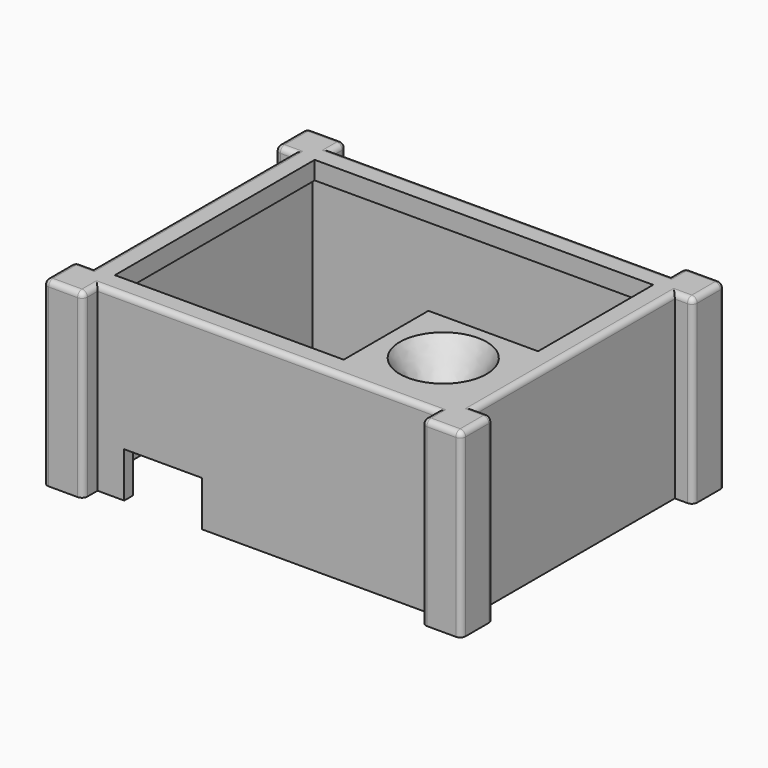
from build123d import *

# Parameters (mm, degrees)
F0_W          = 60.594435811
F0_H          = 58.5138263702
F0_R          = 27.5
F3_DEPTH      = 10
F4_R          = 5
F6_R          = 24
F7_R          = 3
F9_DEPTH      = 10
F10_DEPTH     = 100
F0_W_2        = 42.894218117
F0_H_2        = 6
F11_DEPTH     = 75
F12_R         = 3
F13_T1_DEPTH  = 104.5
F13_S5_W      = 3
F13_S5_H      = 3
F13_T6_DEPTH  = 3
F13_S11_W     = 3
F13_S11_H     = 3
F13_T12_DEPTH = 3
F13_S17_W     = 3
F13_S17_H     = 3
F13_T18_DEPTH = 3
F13_S23_W     = 3
F13_S23_H     = 3
F13_T24_DEPTH = 3
F13_S29_W     = 3
F13_S29_H     = 3
F13_T30_DEPTH = 3
F13_S35_W     = 3
F13_S35_H     = 3
F13_T36_DEPTH = 3
F13_S41_W     = 3
F13_S41_H     = 3
F13_T42_DEPTH = 3
F13_S47_W     = 3
F13_S47_H     = 3
F13_T48_DEPTH = 3
F13_S53_W     = 3
F13_S53_H     = 3
F13_T54_DEPTH = 3
F13_S59_W     = 3
F13_S59_H     = 3
F13_T60_DEPTH = 3
F13_S65_W     = 3
F13_S65_H     = 3
F13_T66_DEPTH = 3
F13_S71_W     = 3
F13_S71_H     = 3
F13_T72_DEPTH = 3
F14_SCALE     = 0.5
F15_ANGLE     = 180


# Not quite as in the source:
# - a fillet or chamfer that OpenCascade refuses, or shapes differently, is made with other operations: its cross-section is extruded or revolved along the edge and cut away or added


with BuildPart() as f3:
    # F0 (on Top) → F3 (new body)
    with BuildSketch(Plane.XY):
        with Locations((162.7266414762, 114.7430868149)):
            Rectangle(F0_W, F0_H)
        with Locations((165, 116)):
            Circle(F0_R, mode=Mode.SUBTRACT)
        with Locations((165, 116)):
            Circle(F0_R)
    extrude(amount=F3_DEPTH)

    # F4 (on offset) → F5 section 0
    with BuildSketch(Plane.XY.offset(36)):
        with Locations((165.0143116713, 116.0647049546)):
            Circle(F4_R)
    # F0 (on Top) → F5 section 1
    with BuildSketch(Plane.XY):
        with Locations((165, 116)):
            Circle(F0_R)
    loft()

    # F6 (on Top) → F8 section 0
    with BuildSketch(Plane.XY):
        with Locations((164.9883985519, 115.9429103136)):
            Circle(F6_R)
    # F7 (on offset) → F8 section 1
    with BuildSketch(Plane.XY.offset(36)):
        with Locations((164.916202426, 116.0804182291)):
            Circle(F7_R)
    loft(mode=Mode.SUBTRACT)

    # F0 (on Top) → F9 (join)
    with BuildSketch(Plane.XY):
        Polygon((0, 150), (0, 0), (199, 0), (199, 150), (63.6303052306, 150), (20.7360871136, 150), align=None)
        Polygon((193.0238593817, 6), (6, 6), (6, 144), (132.4294235706, 144), (193.0238593817, 144), (193.0238593817, 85.4861736298), align=None, mode=Mode.SUBTRACT)
    extrude(amount=F9_DEPTH)

    # F0 (on Top) → F10 (join)
    with BuildSketch(Plane.XY):
        Polygon((199, 0), (0, 0), (0, 150), (20.7360871136, 150), (20.7360871136, 156), (6, 156), (6, 166), (-16, 166), (-16, 144), (-6, 144), (-6, 6), (-16, 6), (-16, -16), (6, -16), (6, -6), (193.0238593817, -6), (193.0238593817, -16), (215, -16), (215, 6), (205, 6), (205, 144), (215, 144), (215, 166), (193.0238593817, 166), (193.0238593817, 156), (63.6303052306, 156), (63.6303052306, 150), (199, 150), align=None)
    extrude(amount=F10_DEPTH)

    # F0 (on Top) → F11 (join)
    with BuildSketch(Plane.XY):
        with Locations((42.1831961721, 153)):
            Rectangle(F0_W_2, F0_H_2)
    extrude(amount=F11_DEPTH)

    # F12
    f12_edges = [f3.edges().sort_by_distance(p)[0] for p in [
        (204.01193, -16, 0),
        (215, -5, 0),
        (205, 75, 0),
        (210, 6, 0),
        (210, 144, 0),
        (215, 155, 0),
        (204.01193, 166, 0),
        (193.023859, 161, 0),
        (99.51193, 156, 0),
        (-5, 166, 0),
        (6, 161, 0),
        (-16, 155, 0),
        (-11, 144, 0),
        (-6, 75, 0),
        (-11, 6, 0),
        (-5, -16, 0),
        (-16, -5, 0),
        (6, -11, 0),
        (99.51193, -6, 0),
        (193.023859, -11, 0),
    ]]
    fillet(f12_edges, radius=F12_R)

    # F13: fillet of radius 3 on 12 edges, made by hand

    # F13_s2 → F13_t1 (cut)
    with BuildSketch(Plane.XY.offset(3)):
        with BuildLine():
            ThreePointArc((212, -16), (214.1213203436, -15.1213203436), (215, -13))
            Line((215, -13), (215, -16))
            Line((215, -16), (212, -16))
        make_face()
        with BuildLine():
            ThreePointArc((193.0238593817, -13), (193.9025390381, -15.1213203436), (196.0238593817, -16))
            Line((196.0238593817, -16), (193.0238593817, -16))
            Line((193.0238593817, -16), (193.0238593817, -13))
        make_face()
        with BuildLine():
            ThreePointArc((215, 3), (214.1213203436, 5.1213203436), (212, 6))
            Line((212, 6), (215, 6))
            Line((215, 6), (215, 3))
        make_face()
        with BuildLine():
            ThreePointArc((212, 144), (214.1213203436, 144.8786796564), (215, 147))
            Line((215, 147), (215, 144))
            Line((215, 144), (212, 144))
        make_face()
        with BuildLine():
            ThreePointArc((215, 163), (214.1213203436, 165.1213203436), (212, 166))
            Line((212, 166), (215, 166))
            Line((215, 166), (215, 163))
        make_face()
        with BuildLine():
            ThreePointArc((193.0238593817, 163), (193.9025390381, 165.1213203436), (196.0238593817, 166))
            Line((196.0238593817, 166), (193.0238593817, 166))
            Line((193.0238593817, 166), (193.0238593817, 163))
        make_face()
        with BuildLine():
            ThreePointArc((3, -16), (5.1213203436, -15.1213203436), (6, -13))
            Line((6, -13), (6, -16))
            Line((6, -16), (3, -16))
        make_face()
        with BuildLine():
            ThreePointArc((-16, -13), (-15.1213203436, -15.1213203436), (-13, -16))
            Line((-13, -16), (-16, -16))
            Line((-16, -16), (-16, -13))
        make_face()
        with BuildLine():
            ThreePointArc((-13, 6), (-15.1213203436, 5.1213203436), (-16, 3))
            Line((-16, 3), (-16, 6))
            Line((-16, 6), (-13, 6))
        make_face()
        with BuildLine():
            ThreePointArc((-16, 147), (-15.1213203436, 144.8786796564), (-13, 144))
            Line((-13, 144), (-16, 144))
            Line((-16, 144), (-16, 147))
        make_face()
        with BuildLine():
            ThreePointArc((-13, 166), (-15.1213203436, 165.1213203436), (-16, 163))
            Line((-16, 163), (-16, 166))
            Line((-16, 166), (-13, 166))
        make_face()
        with BuildLine():
            ThreePointArc((6, 163), (5.1213203436, 165.1213203436), (3, 166))
            Line((3, 166), (6, 166))
            Line((6, 166), (6, 163))
        make_face()
    extrude(amount=F13_T1_DEPTH, mode=Mode.SUBTRACT)


with BuildPart() as f13_tool4:
    # F13_s5 → F13_t6 (new body)
    with BuildSketch(Plane.YZ.offset(3)):
        with Locations((164.5, 1.5)):
            Rectangle(F13_S5_W, F13_S5_H)
    extrude(amount=F13_T6_DEPTH)

    # F13_s7 → F13_t8 (revolve, cut)
    with BuildSketch(Plane(origin=(3, 163, 3), x_dir=(0, -0.7071067812, 0.7071067812), z_dir=(0, 0.7071067812, 0.7071067812))):
        with BuildLine():
            ThreePointArc((0, -3), (3, 0), (0, 3))
            Line((0, 3), (0, -3))
        make_face()
    revolve(axis=Axis((3, 163, 3), (1, 0, 0)), mode=Mode.SUBTRACT)


with BuildPart() as f3_1:
    add(f3.part)

    # F13_t3: cut F13_tool4
    add(f13_tool4.part, mode=Mode.SUBTRACT)


with BuildPart() as f13_tool10:
    # F13_s11 → F13_t12 (new body)
    with BuildSketch(Plane.XZ.offset(-163)):
        with Locations((-14.5, 1.5)):
            Rectangle(F13_S11_W, F13_S11_H)
    extrude(amount=-F13_T12_DEPTH)

    # F13_s13 → F13_t14 (revolve, cut)
    with BuildSketch(Plane(origin=(-13, 163, 3), x_dir=(0.7071067812, 0, 0.7071067812), z_dir=(-0.7071067812, 0, 0.7071067812))):
        with BuildLine():
            ThreePointArc((0, -3), (3, 0), (0, 3))
            Line((0, 3), (0, -3))
        make_face()
    revolve(axis=Axis((-13, 163, 3), (0, 1, 0)), mode=Mode.SUBTRACT)


with BuildPart() as f3_2:
    add(f3_1.part)

    # F13_t9: cut F13_tool10
    add(f13_tool10.part, mode=Mode.SUBTRACT)


with BuildPart() as f13_tool16:
    # F13_s17 → F13_t18 (new body)
    with BuildSketch(Plane.YZ.offset(-13)):
        with Locations((145.5, 1.5)):
            Rectangle(F13_S17_W, F13_S17_H)
    extrude(amount=-F13_T18_DEPTH)

    # F13_s19 → F13_t20 (revolve, cut)
    with BuildSketch(Plane(origin=(-13, 147, 3), x_dir=(0, 0.7071067812, 0.7071067812), z_dir=(0, -0.7071067812, 0.7071067812))):
        with BuildLine():
            ThreePointArc((0, -3), (3, 0), (0, 3))
            Line((0, 3), (0, -3))
        make_face()
    revolve(axis=Axis((-13, 147, 3), (-1, 0, 0)), mode=Mode.SUBTRACT)


with BuildPart() as f3_3:
    add(f3_2.part)

    # F13_t15: cut F13_tool16
    add(f13_tool16.part, mode=Mode.SUBTRACT)


with BuildPart() as f13_tool22:
    # F13_s23 → F13_t24 (new body)
    with BuildSketch(Plane.XZ.offset(-3)):
        with Locations((-14.5, 1.5)):
            Rectangle(F13_S23_W, F13_S23_H)
    extrude(amount=-F13_T24_DEPTH)

    # F13_s25 → F13_t26 (revolve, cut)
    with BuildSketch(Plane(origin=(-13, 3, 3), x_dir=(0.7071067812, 0, 0.7071067812), z_dir=(-0.7071067812, 0, 0.7071067812))):
        with BuildLine():
            ThreePointArc((0, -3), (3, 0), (0, 3))
            Line((0, 3), (0, -3))
        make_face()
    revolve(axis=Axis((-13, 3, 3), (0, 1, 0)), mode=Mode.SUBTRACT)


with BuildPart() as f3_4:
    add(f3_3.part)

    # F13_t21: cut F13_tool22
    add(f13_tool22.part, mode=Mode.SUBTRACT)


with BuildPart() as f13_tool28:
    # F13_s29 → F13_t30 (new body)
    with BuildSketch(Plane.YZ.offset(-13)):
        with Locations((-14.5, 1.5)):
            Rectangle(F13_S29_W, F13_S29_H)
    extrude(amount=-F13_T30_DEPTH)

    # F13_s31 → F13_t32 (revolve, cut)
    with BuildSketch(Plane(origin=(-13, -13, 3), x_dir=(0, 0.7071067812, 0.7071067812), z_dir=(0, -0.7071067812, 0.7071067812))):
        with BuildLine():
            ThreePointArc((0, -3), (3, 0), (0, 3))
            Line((0, 3), (0, -3))
        make_face()
    revolve(axis=Axis((-13, -13, 3), (-1, 0, 0)), mode=Mode.SUBTRACT)


with BuildPart() as f3_5:
    add(f3_4.part)

    # F13_t27: cut F13_tool28
    add(f13_tool28.part, mode=Mode.SUBTRACT)


with BuildPart() as f13_tool34:
    # F13_s35 → F13_t36 (new body)
    with BuildSketch(Plane.XZ.offset(13)):
        with Locations((4.5, 1.5)):
            Rectangle(F13_S35_W, F13_S35_H)
    extrude(amount=F13_T36_DEPTH)

    # F13_s37 → F13_t38 (revolve, cut)
    with BuildSketch(Plane(origin=(3, -13, 3), x_dir=(-0.7071067812, 0, 0.7071067812), z_dir=(0.7071067812, 0, 0.7071067812))):
        with BuildLine():
            ThreePointArc((0, -3), (3, 0), (0, 3))
            Line((0, 3), (0, -3))
        make_face()
    revolve(axis=Axis((3, -13, 3), (0, -1, 0)), mode=Mode.SUBTRACT)


with BuildPart() as f3_6:
    add(f3_5.part)

    # F13_t33: cut F13_tool34
    add(f13_tool34.part, mode=Mode.SUBTRACT)


with BuildPart() as f13_tool40:
    # F13_s41 → F13_t42 (new body)
    with BuildSketch(Plane.YZ.offset(196.0238593817)):
        with Locations((164.5, 1.5)):
            Rectangle(F13_S41_W, F13_S41_H)
    extrude(amount=-F13_T42_DEPTH)

    # F13_s43 → F13_t44 (revolve, cut)
    with BuildSketch(Plane(origin=(196.0238593817, 163, 3), x_dir=(0, -0.7071067812, 0.7071067812), z_dir=(0, -0.7071067812, -0.7071067812))):
        with BuildLine():
            ThreePointArc((0, -3), (3, 0), (0, 3))
            Line((0, 3), (0, -3))
        make_face()
    revolve(axis=Axis((196.0238593817, 163, 3), (-1, 0, 0)), mode=Mode.SUBTRACT)


with BuildPart() as f3_7:
    add(f3_6.part)

    # F13_t39: cut F13_tool40
    add(f13_tool40.part, mode=Mode.SUBTRACT)


with BuildPart() as f13_tool46:
    # F13_s47 → F13_t48 (new body)
    with BuildSketch(Plane.YZ.offset(212)):
        with Locations((164.5, 1.5)):
            Rectangle(F13_S47_W, F13_S47_H)
    extrude(amount=F13_T48_DEPTH)

    # F13_s49 → F13_t50 (revolve, cut)
    with BuildSketch(Plane(origin=(212, 163, 3), x_dir=(0, -0.7071067812, 0.7071067812), z_dir=(0, 0.7071067812, 0.7071067812))):
        with BuildLine():
            ThreePointArc((0, -3), (3, 0), (0, 3))
            Line((0, 3), (0, -3))
        make_face()
    revolve(axis=Axis((212, 163, 3), (1, 0, 0)), mode=Mode.SUBTRACT)


with BuildPart() as f3_8:
    add(f3_7.part)

    # F13_t45: cut F13_tool46
    add(f13_tool46.part, mode=Mode.SUBTRACT)


with BuildPart() as f13_tool52:
    # F13_s53 → F13_t54 (new body)
    with BuildSketch(Plane.XZ.offset(-147)):
        with Locations((213.5, 1.5)):
            Rectangle(F13_S53_W, F13_S53_H)
    extrude(amount=F13_T54_DEPTH)

    # F13_s55 → F13_t56 (revolve, cut)
    with BuildSketch(Plane(origin=(212, 147, 3), x_dir=(-0.7071067812, 0, 0.7071067812), z_dir=(0.7071067812, 0, 0.7071067812))):
        with BuildLine():
            ThreePointArc((0, -3), (3, 0), (0, 3))
            Line((0, 3), (0, -3))
        make_face()
    revolve(axis=Axis((212, 147, 3), (0, -1, 0)), mode=Mode.SUBTRACT)


with BuildPart() as f3_9:
    add(f3_8.part)

    # F13_t51: cut F13_tool52
    add(f13_tool52.part, mode=Mode.SUBTRACT)


with BuildPart() as f13_tool58:
    # F13_s59 → F13_t60 (new body)
    with BuildSketch(Plane.YZ.offset(212)):
        with Locations((4.5, 1.5)):
            Rectangle(F13_S59_W, F13_S59_H)
    extrude(amount=F13_T60_DEPTH)

    # F13_s61 → F13_t62 (revolve, cut)
    with BuildSketch(Plane(origin=(212, 3, 3), x_dir=(0, -0.7071067812, 0.7071067812), z_dir=(0, 0.7071067812, 0.7071067812))):
        with BuildLine():
            ThreePointArc((0, -3), (3, 0), (0, 3))
            Line((0, 3), (0, -3))
        make_face()
    revolve(axis=Axis((212, 3, 3), (1, 0, 0)), mode=Mode.SUBTRACT)


with BuildPart() as f3_10:
    add(f3_9.part)

    # F13_t57: cut F13_tool58
    add(f13_tool58.part, mode=Mode.SUBTRACT)


with BuildPart() as f13_tool64:
    # F13_s65 → F13_t66 (new body)
    with BuildSketch(Plane.YZ.offset(196.0238593817)):
        with Locations((-14.5, 1.5)):
            Rectangle(F13_S65_W, F13_S65_H)
    extrude(amount=-F13_T66_DEPTH)

    # F13_s67 → F13_t68 (revolve, cut)
    with BuildSketch(Plane(origin=(196.0238593817, -13, 3), x_dir=(0, 0.7071067812, 0.7071067812), z_dir=(0, -0.7071067812, 0.7071067812))):
        with BuildLine():
            ThreePointArc((0, -3), (3, 0), (0, 3))
            Line((0, 3), (0, -3))
        make_face()
    revolve(axis=Axis((196.0238593817, -13, 3), (-1, 0, 0)), mode=Mode.SUBTRACT)


with BuildPart() as f3_11:
    add(f3_10.part)

    # F13_t63: cut F13_tool64
    add(f13_tool64.part, mode=Mode.SUBTRACT)


with BuildPart() as f13_tool70:
    # F13_s71 → F13_t72 (new body)
    with BuildSketch(Plane.XZ.offset(13)):
        with Locations((213.5, 1.5)):
            Rectangle(F13_S71_W, F13_S71_H)
    extrude(amount=F13_T72_DEPTH)

    # F13_s73 → F13_t74 (revolve, cut)
    with BuildSketch(Plane(origin=(212, -13, 3), x_dir=(-0.7071067812, 0, 0.7071067812), z_dir=(0.7071067812, 0, 0.7071067812))):
        with BuildLine():
            ThreePointArc((0, -3), (3, 0), (0, 3))
            Line((0, 3), (0, -3))
        make_face()
    revolve(axis=Axis((212, -13, 3), (0, -1, 0)), mode=Mode.SUBTRACT)


with BuildPart() as f3_12:
    add(f3_11.part)

    # F13_t69: cut F13_tool70
    add(f13_tool70.part, mode=Mode.SUBTRACT)


with BuildPart() as f3_13:
    # F14: moved
    add(f3_12.part.scale(F14_SCALE).moved(Location((107.5, -8, 0))))


with BuildPart() as f3_14:
    # F15: moved
    add(f3_13.part.rotate(Axis((99.5119296908, -6, 0), (1, 0, 0)), F15_ANGLE))


solid = f3_14.part
